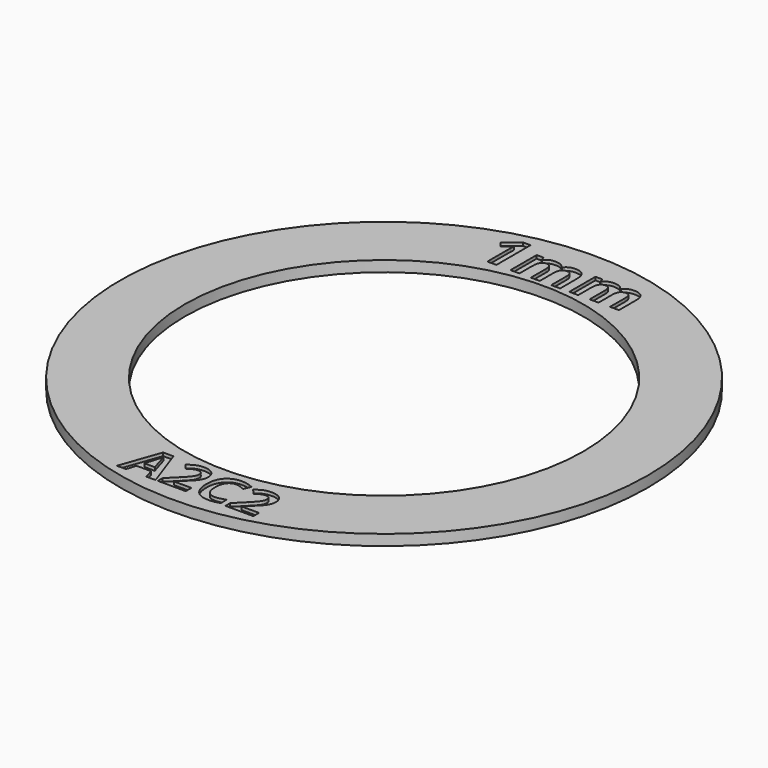
from build123d import *

# Parameters (mm, degrees)
F0_R           = 24.5
F0_R_2         = 18.5
F0_TEXT_SIZE   = 5.1974965673
F0_TEXT_SIZE_2 = 5.5555555556
F1_DEPTH       = 1
F2_DEPTH       = 0.3


# Not quite as in the source:
# - Text() gives the source's letters only with a copy of the font that has no kerning and outlines rounded to 1/6400 em; it was checked with that copy


with BuildPart() as f1:
    # F0 (on Top) → F1 (new body)
    with BuildSketch(Plane.XY):
        Circle(F0_R)
        Polygon((-2.9154707307, -22.8730905801), (-3.7633123583, -22.8730905801), (-4.0321203839, -21.9895161637), (-5.3850937091, -21.9895161637), (-5.6539017347, -22.8730905801), (-6.5017433622, -22.8730905801), (-5.1918118055, -19.1471352284), (-4.2302749405, -19.1471352284), align=None, mode=Mode.SUBTRACT)
        with BuildLine():
            Line((-0.1136952374, -22.2128460943), (-0.1136952374, -22.8730905801))
            Line((-0.1136952374, -22.8730905801), (-2.707570868, -22.8730905801))
            Line((-2.707570868, -22.8730905801), (-2.707570868, -22.3273534405))
            Line((-2.707570868, -22.3273534405), (-1.7760820301, -21.3861192965))
            add(Edge.make_bspline(
                [(-1.7760820301, -21.3861192965), (-1.3619065224, -20.9621984828), (-1.2352175436, -20.7985585518)],
                knots=[0, 0, 0, 1, 1, 1], degree=2))
            add(Edge.make_bspline(
                [(-1.2352175436, -20.7985585518), (-1.1085285648, -20.6349186208), (-1.0524930549, -20.4952359005)],
                knots=[0, 0, 0, 1, 1, 1], degree=2))
            add(Edge.make_bspline(
                [(-1.0524930549, -20.4952359005), (-0.996457545, -20.3555531803), (-0.996457545, -20.206125154)],
                knots=[0, 0, 0, 1, 1, 1], degree=2))
            add(Edge.make_bspline(
                [(-0.996457545, -20.206125154), (-0.996457545, -19.9827952234), (-1.1198980885, -19.8735665846)],
                knots=[0, 0, 0, 1, 1, 1], degree=2))
            add(Edge.make_bspline(
                [(-1.1198980885, -19.8735665846), (-1.243338632, -19.7643379458), (-1.4488021681, -19.7643379458)],
                knots=[0, 0, 0, 1, 1, 1], degree=2))
            add(Edge.make_bspline(
                [(-1.4488021681, -19.7643379458), (-1.6640110104, -19.7643379458), (-1.86703822, -19.8634152241)],
                knots=[0, 0, 0, 1, 1, 1], degree=2))
            add(Edge.make_bspline(
                [(-1.86703822, -19.8634152241), (-2.0700654297, -19.9624925024), (-2.2909590338, -20.1452169911)],
                knots=[0, 0, 0, 1, 1, 1], degree=2))
            Line((-2.2909590338, -20.1452169911), (-2.7173161741, -19.6400852935))
            add(Edge.make_bspline(
                [(-2.7173161741, -19.6400852935), (-2.4436354955, -19.4061979479), (-2.2633473333, -19.3099630505)],
                knots=[0, 0, 0, 1, 1, 1], degree=2))
            add(Edge.make_bspline(
                [(-2.2633473333, -19.3099630505), (-2.0830591711, -19.2137281532), (-1.869880601, -19.1617531875)],
                knots=[0, 0, 0, 1, 1, 1], degree=2))
            add(Edge.make_bspline(
                [(-1.869880601, -19.1617531875), (-1.6567020308, -19.1097782218), (-1.3927666583, -19.1097782218)],
                knots=[0, 0, 0, 1, 1, 1], degree=2))
            add(Edge.make_bspline(
                [(-1.3927666583, -19.1097782218), (-1.0451840753, -19.1097782218), (-0.7788123763, -19.2364672006)],
                knots=[0, 0, 0, 1, 1, 1], degree=2))
            add(Edge.make_bspline(
                [(-0.7788123763, -19.2364672006), (-0.5124406772, -19.3631561795), (-0.365042923, -19.5917648176)],
                knots=[0, 0, 0, 1, 1, 1], degree=2))
            add(Edge.make_bspline(
                [(-0.365042923, -19.5917648176), (-0.2176451688, -19.8203734556), (-0.2176451688, -20.1143568552)],
                knots=[0, 0, 0, 1, 1, 1], degree=2))
            add(Edge.make_bspline(
                [(-0.2176451688, -20.1143568552), (-0.2176451688, -20.3709832482), (-0.3077892498, -20.5955313421)],
                knots=[0, 0, 0, 1, 1, 1], degree=2))
            add(Edge.make_bspline(
                [(-0.3077892498, -20.5955313421), (-0.3979333309, -20.820079436), (-0.5871546903, -21.0559970536)],
                knots=[0, 0, 0, 1, 1, 1], degree=2))
            add(Edge.make_bspline(
                [(-0.5871546903, -21.0559970536), (-0.7763760497, -21.2919146713), (-1.253083938, -21.7288292265)],
                knots=[0, 0, 0, 1, 1, 1], degree=2))
            Line((-1.253083938, -21.7288292265), (-1.7306039352, -22.1779254142))
            Line((-1.7306039352, -22.1779254142), (-1.7306039352, -22.2128460943))
            Line((-1.7306039352, -22.2128460943), (-0.1136952374, -22.2128460943))
        make_face(mode=Mode.SUBTRACT)
        Circle(F0_R_2, mode=Mode.SUBTRACT)
        with BuildLine():
            add(Edge.make_bspline(
                [(2.5077920937, -19.8378337957), (2.2974559045, -19.7643379458), (2.0944286949, -19.7643379458)],
                knots=[0, 0, 0, 1, 1, 1], degree=2))
            add(Edge.make_bspline(
                [(2.0944286949, -19.7643379458), (1.6502051601, -19.7643379458), (1.4065725085, -20.0981146785)],
                knots=[0, 0, 0, 1, 1, 1], degree=2))
            add(Edge.make_bspline(
                [(1.4065725085, -20.0981146785), (1.1629398569, -20.4318914111), (1.1629398569, -21.0279792987)],
                knots=[0, 0, 0, 1, 1, 1], degree=2))
            add(Edge.make_bspline(
                [(1.1629398569, -21.0279792987), (1.1629398569, -22.2688816042), (2.0944286949, -22.2688816042)],
                knots=[0, 0, 0, 1, 1, 1], degree=2))
            add(Edge.make_bspline(
                [(2.0944286949, -22.2688816042), (2.4850530463, -22.2688816042), (3.0405354919, -22.0739754829)],
                knots=[0, 0, 0, 1, 1, 1], degree=2))
            Line((3.0405354919, -22.0739754829), (3.0405354919, -22.7334078599))
            add(Edge.make_bspline(
                [(3.0405354919, -22.7334078599), (2.5841303246, -22.9242534369), (2.0205267906, -22.9242534369)],
                knots=[0, 0, 0, 1, 1, 1], degree=2))
            add(Edge.make_bspline(
                [(2.0205267906, -22.9242534369), (1.2108542784, -22.9242534369), (0.7820608116, -22.4329275896)],
                knots=[0, 0, 0, 1, 1, 1], degree=2))
            add(Edge.make_bspline(
                [(0.7820608116, -22.4329275896), (0.3532673448, -21.9416017422), (0.3532673448, -21.0231066457)],
                knots=[0, 0, 0, 1, 1, 1], degree=2))
            add(Edge.make_bspline(
                [(0.3532673448, -21.0231066457), (0.3532673448, -20.4440730437), (0.5640095884, -20.0087827062)],
                knots=[0, 0, 0, 1, 1, 1], degree=2))
            add(Edge.make_bspline(
                [(0.5640095884, -20.0087827062), (0.7747518321, -19.5734923687), (1.1694367277, -19.3416352953)],
                knots=[0, 0, 0, 1, 1, 1], degree=2))
            add(Edge.make_bspline(
                [(1.1694367277, -19.3416352953), (1.5641216232, -19.1097782218), (2.0944286949, -19.1097782218)],
                knots=[0, 0, 0, 1, 1, 1], degree=2))
            add(Edge.make_bspline(
                [(2.0944286949, -19.1097782218), (2.6344810726, -19.1097782218), (3.1802182121, -19.370465159)],
                knots=[0, 0, 0, 1, 1, 1], degree=2))
            Line((3.1802182121, -19.370465159), (2.9268402545, -20.0104069239))
            add(Edge.make_bspline(
                [(2.9268402545, -20.0104069239), (2.7181282829, -19.9113296456), (2.5077920937, -19.8378337957)],
                knots=[0, 0, 0, 1, 1, 1], degree=2))
        make_face(mode=Mode.SUBTRACT)
        with BuildLine():
            Line((6.1647181942, -22.2128460943), (6.1647181942, -22.8730905801))
            Line((6.1647181942, -22.8730905801), (3.5708425635, -22.8730905801))
            Line((3.5708425635, -22.8730905801), (3.5708425635, -22.3273534405))
            Line((3.5708425635, -22.3273534405), (4.5023314015, -21.3861192965))
            add(Edge.make_bspline(
                [(4.5023314015, -21.3861192965), (4.9165069092, -20.9621984828), (5.043195888, -20.7985585518)],
                knots=[0, 0, 0, 1, 1, 1], degree=2))
            add(Edge.make_bspline(
                [(5.043195888, -20.7985585518), (5.1698848668, -20.6349186208), (5.2259203767, -20.4952359005)],
                knots=[0, 0, 0, 1, 1, 1], degree=2))
            add(Edge.make_bspline(
                [(5.2259203767, -20.4952359005), (5.2819558866, -20.3555531803), (5.2819558866, -20.206125154)],
                knots=[0, 0, 0, 1, 1, 1], degree=2))
            add(Edge.make_bspline(
                [(5.2819558866, -20.206125154), (5.2819558866, -19.9827952234), (5.1585153431, -19.8735665846)],
                knots=[0, 0, 0, 1, 1, 1], degree=2))
            add(Edge.make_bspline(
                [(5.1585153431, -19.8735665846), (5.0350747996, -19.7643379458), (4.8296112634, -19.7643379458)],
                knots=[0, 0, 0, 1, 1, 1], degree=2))
            add(Edge.make_bspline(
                [(4.8296112634, -19.7643379458), (4.6144024212, -19.7643379458), (4.4113752115, -19.8634152241)],
                knots=[0, 0, 0, 1, 1, 1], degree=2))
            add(Edge.make_bspline(
                [(4.4113752115, -19.8634152241), (4.2083480019, -19.9624925024), (3.9874543978, -20.1452169911)],
                knots=[0, 0, 0, 1, 1, 1], degree=2))
            Line((3.9874543978, -20.1452169911), (3.5610972575, -19.6400852935))
            add(Edge.make_bspline(
                [(3.5610972575, -19.6400852935), (3.8347779361, -19.4061979479), (4.0150660983, -19.3099630505)],
                knots=[0, 0, 0, 1, 1, 1], degree=2))
            add(Edge.make_bspline(
                [(4.0150660983, -19.3099630505), (4.1953542604, -19.2137281532), (4.4085328306, -19.1617531875)],
                knots=[0, 0, 0, 1, 1, 1], degree=2))
            add(Edge.make_bspline(
                [(4.4085328306, -19.1617531875), (4.6217114007, -19.1097782218), (4.8856467733, -19.1097782218)],
                knots=[0, 0, 0, 1, 1, 1], degree=2))
            add(Edge.make_bspline(
                [(4.8856467733, -19.1097782218), (5.2332293562, -19.1097782218), (5.4996010553, -19.2364672006)],
                knots=[0, 0, 0, 1, 1, 1], degree=2))
            add(Edge.make_bspline(
                [(5.4996010553, -19.2364672006), (5.7659727544, -19.3631561795), (5.9133705086, -19.5917648176)],
                knots=[0, 0, 0, 1, 1, 1], degree=2))
            add(Edge.make_bspline(
                [(5.9133705086, -19.5917648176), (6.0607682628, -19.8203734556), (6.0607682628, -20.1143568552)],
                knots=[0, 0, 0, 1, 1, 1], degree=2))
            add(Edge.make_bspline(
                [(6.0607682628, -20.1143568552), (6.0607682628, -20.3709832482), (5.9706241817, -20.5955313421)],
                knots=[0, 0, 0, 1, 1, 1], degree=2))
            add(Edge.make_bspline(
                [(5.9706241817, -20.5955313421), (5.8804801006, -20.820079436), (5.6912587412, -21.0559970536)],
                knots=[0, 0, 0, 1, 1, 1], degree=2))
            add(Edge.make_bspline(
                [(5.6912587412, -21.0559970536), (5.5020373818, -21.2919146713), (5.0253294935, -21.7288292265)],
                knots=[0, 0, 0, 1, 1, 1], degree=2))
            Line((5.0253294935, -21.7288292265), (4.5478094964, -22.1779254142))
            Line((4.5478094964, -22.1779254142), (4.5478094964, -22.2128460943))
            Line((4.5478094964, -22.2128460943), (6.1647181942, -22.2128460943))
        make_face(mode=Mode.SUBTRACT)
        with BuildLine():
            Line((-4.7178819444, 22.8950881169), (-4.7178819444, 18.9289422836))
            Line((-4.7178819444, 18.9289422836), (-5.5564236111, 18.9289422836))
            Line((-5.5564236111, 18.9289422836), (-5.5564236111, 21.2240811725))
            Line((-5.5564236111, 21.2240811725), (-5.5477430556, 21.6008172836))
            Line((-5.5477430556, 21.6008172836), (-5.5347222222, 22.0131436725))
            add(Edge.make_bspline(
                [(-5.5347222222, 22.0131436725), (-5.7430555556, 21.8048103392), (-5.8246527778, 21.7397061725)],
                knots=[0, 0, 0, 1, 1, 1], degree=2))
            Line((-5.8246527778, 21.7397061725), (-6.2803819444, 21.3733867281))
            Line((-6.2803819444, 21.3733867281), (-6.6848958333, 21.8777270058))
            Line((-6.6848958333, 21.8777270058), (-5.4071180556, 22.8950881169))
            Line((-5.4071180556, 22.8950881169), (-4.7178819444, 22.8950881169))
        make_face(mode=Mode.SUBTRACT)
        with BuildLine():
            Line((-0.6927083333, 20.4506436725), (-0.6927083333, 18.9289422836))
            Line((-0.6927083333, 18.9289422836), (-1.5199652778, 18.9289422836))
            Line((-1.5199652778, 18.9289422836), (-1.5199652778, 20.7006436725))
            add(Edge.make_bspline(
                [(-1.5199652778, 20.7006436725), (-1.5199652778, 21.0287686725), (-1.6297743056, 21.1928311725)],
                knots=[0, 0, 0, 1, 1, 1], degree=2))
            add(Edge.make_bspline(
                [(-1.6297743056, 21.1928311725), (-1.7395833333, 21.3568936725), (-1.9756944444, 21.3568936725)],
                knots=[0, 0, 0, 1, 1, 1], degree=2))
            add(Edge.make_bspline(
                [(-1.9756944444, 21.3568936725), (-2.2934027778, 21.3568936725), (-2.4370659722, 21.1233867281)],
                knots=[0, 0, 0, 1, 1, 1], degree=2))
            add(Edge.make_bspline(
                [(-2.4370659722, 21.1233867281), (-2.5807291667, 20.8898797836), (-2.5807291667, 20.3560256169)],
                knots=[0, 0, 0, 1, 1, 1], degree=2))
            Line((-2.5807291667, 20.3560256169), (-2.5807291667, 18.9289422836))
            Line((-2.5807291667, 18.9289422836), (-3.4079861111, 18.9289422836))
            Line((-3.4079861111, 18.9289422836), (-3.4079861111, 21.9619283947))
            Line((-3.4079861111, 21.9619283947), (-2.7760416667, 21.9619283947))
            Line((-2.7760416667, 21.9619283947), (-2.6649305556, 21.5739075614))
            Line((-2.6649305556, 21.5739075614), (-2.6189236111, 21.5739075614))
            add(Edge.make_bspline(
                [(-2.6189236111, 21.5739075614), (-2.4965277778, 21.7831089503), (-2.2660590278, 21.9007304781)],
                knots=[0, 0, 0, 1, 1, 1], degree=2))
            add(Edge.make_bspline(
                [(-2.2660590278, 21.9007304781), (-2.0355902778, 22.0183520058), (-1.7369791667, 22.0183520058)],
                knots=[0, 0, 0, 1, 1, 1], degree=2))
            add(Edge.make_bspline(
                [(-1.7369791667, 22.0183520058), (-1.0564236111, 22.0183520058), (-0.8142361111, 21.5739075614)],
                knots=[0, 0, 0, 1, 1, 1], degree=2))
            Line((-0.8142361111, 21.5739075614), (-0.7413194444, 21.5739075614))
            add(Edge.make_bspline(
                [(-0.7413194444, 21.5739075614), (-0.6189236111, 21.7857131169), (-0.3819444444, 21.9020325614)],
                knots=[0, 0, 0, 1, 1, 1], degree=2))
            add(Edge.make_bspline(
                [(-0.3819444444, 21.9020325614), (-0.1449652778, 22.0183520058), (0.1536458333, 22.0183520058)],
                knots=[0, 0, 0, 1, 1, 1], degree=2))
            add(Edge.make_bspline(
                [(0.1536458333, 22.0183520058), (0.6692708333, 22.0183520058), (0.93359375, 21.7540290892)],
                knots=[0, 0, 0, 1, 1, 1], degree=2))
            add(Edge.make_bspline(
                [(0.93359375, 21.7540290892), (1.1979166667, 21.4897061725), (1.1979166667, 20.9063728392)],
                knots=[0, 0, 0, 1, 1, 1], degree=2))
            Line((1.1979166667, 20.9063728392), (1.1979166667, 18.9289422836))
            Line((1.1979166667, 18.9289422836), (0.3680555556, 18.9289422836))
            Line((0.3680555556, 18.9289422836), (0.3680555556, 20.7006436725))
            add(Edge.make_bspline(
                [(0.3680555556, 20.7006436725), (0.3680555556, 21.0287686725), (0.2582465278, 21.1928311725)],
                knots=[0, 0, 0, 1, 1, 1], degree=2))
            add(Edge.make_bspline(
                [(0.2582465278, 21.1928311725), (0.1484375, 21.3568936725), (-0.0876736111, 21.3568936725)],
                knots=[0, 0, 0, 1, 1, 1], degree=2))
            add(Edge.make_bspline(
                [(-0.0876736111, 21.3568936725), (-0.3914930556, 21.3568936725), (-0.5421006944, 21.1398797836)],
                knots=[0, 0, 0, 1, 1, 1], degree=2))
            add(Edge.make_bspline(
                [(-0.5421006944, 21.1398797836), (-0.6927083333, 20.9228658947), (-0.6927083333, 20.4506436725)],
                knots=[0, 0, 0, 1, 1, 1], degree=2))
        make_face(mode=Mode.SUBTRACT)
        with BuildLine():
            Line((4.7621527778, 20.4506436725), (4.7621527778, 18.9289422836))
            Line((4.7621527778, 18.9289422836), (3.9348958333, 18.9289422836))
            Line((3.9348958333, 18.9289422836), (3.9348958333, 20.7006436725))
            add(Edge.make_bspline(
                [(3.9348958333, 20.7006436725), (3.9348958333, 21.0287686725), (3.8250868056, 21.1928311725)],
                knots=[0, 0, 0, 1, 1, 1], degree=2))
            add(Edge.make_bspline(
                [(3.8250868056, 21.1928311725), (3.7152777778, 21.3568936725), (3.4791666667, 21.3568936725)],
                knots=[0, 0, 0, 1, 1, 1], degree=2))
            add(Edge.make_bspline(
                [(3.4791666667, 21.3568936725), (3.1614583333, 21.3568936725), (3.0177951389, 21.1233867281)],
                knots=[0, 0, 0, 1, 1, 1], degree=2))
            add(Edge.make_bspline(
                [(3.0177951389, 21.1233867281), (2.8741319444, 20.8898797836), (2.8741319444, 20.3560256169)],
                knots=[0, 0, 0, 1, 1, 1], degree=2))
            Line((2.8741319444, 20.3560256169), (2.8741319444, 18.9289422836))
            Line((2.8741319444, 18.9289422836), (2.046875, 18.9289422836))
            Line((2.046875, 18.9289422836), (2.046875, 21.9619283947))
            Line((2.046875, 21.9619283947), (2.6788194444, 21.9619283947))
            Line((2.6788194444, 21.9619283947), (2.7899305556, 21.5739075614))
            Line((2.7899305556, 21.5739075614), (2.8359375, 21.5739075614))
            add(Edge.make_bspline(
                [(2.8359375, 21.5739075614), (2.9583333333, 21.7831089503), (3.1888020833, 21.9007304781)],
                knots=[0, 0, 0, 1, 1, 1], degree=2))
            add(Edge.make_bspline(
                [(3.1888020833, 21.9007304781), (3.4192708333, 22.0183520058), (3.7178819444, 22.0183520058)],
                knots=[0, 0, 0, 1, 1, 1], degree=2))
            add(Edge.make_bspline(
                [(3.7178819444, 22.0183520058), (4.3984375, 22.0183520058), (4.640625, 21.5739075614)],
                knots=[0, 0, 0, 1, 1, 1], degree=2))
            Line((4.640625, 21.5739075614), (4.7135416667, 21.5739075614))
            add(Edge.make_bspline(
                [(4.7135416667, 21.5739075614), (4.8359375, 21.7857131169), (5.0729166667, 21.9020325614)],
                knots=[0, 0, 0, 1, 1, 1], degree=2))
            add(Edge.make_bspline(
                [(5.0729166667, 21.9020325614), (5.3098958333, 22.0183520058), (5.6085069444, 22.0183520058)],
                knots=[0, 0, 0, 1, 1, 1], degree=2))
            add(Edge.make_bspline(
                [(5.6085069444, 22.0183520058), (6.1241319444, 22.0183520058), (6.3884548611, 21.7540290892)],
                knots=[0, 0, 0, 1, 1, 1], degree=2))
            add(Edge.make_bspline(
                [(6.3884548611, 21.7540290892), (6.6527777778, 21.4897061725), (6.6527777778, 20.9063728392)],
                knots=[0, 0, 0, 1, 1, 1], degree=2))
            Line((6.6527777778, 20.9063728392), (6.6527777778, 18.9289422836))
            Line((6.6527777778, 18.9289422836), (5.8229166667, 18.9289422836))
            Line((5.8229166667, 18.9289422836), (5.8229166667, 20.7006436725))
            add(Edge.make_bspline(
                [(5.8229166667, 20.7006436725), (5.8229166667, 21.0287686725), (5.7131076389, 21.1928311725)],
                knots=[0, 0, 0, 1, 1, 1], degree=2))
            add(Edge.make_bspline(
                [(5.7131076389, 21.1928311725), (5.6032986111, 21.3568936725), (5.3671875, 21.3568936725)],
                knots=[0, 0, 0, 1, 1, 1], degree=2))
            add(Edge.make_bspline(
                [(5.3671875, 21.3568936725), (5.0633680556, 21.3568936725), (4.9127604167, 21.1398797836)],
                knots=[0, 0, 0, 1, 1, 1], degree=2))
            add(Edge.make_bspline(
                [(4.9127604167, 21.1398797836), (4.7621527778, 20.9228658947), (4.7621527778, 20.4506436725)],
                knots=[0, 0, 0, 1, 1, 1], degree=2))
        make_face(mode=Mode.SUBTRACT)
        with Locations((-6.5017433622, -22.8730905801)):
            Text('A2C2', F0_TEXT_SIZE, font='Open Sans', font_style=FontStyle.BOLD, text_align=(TextAlign.LEFT, TextAlign.BOTTOM))
        with Locations((-7.0130208333, 18.9289422836)):
            Text('1mm', F0_TEXT_SIZE_2, font='Open Sans', font_style=FontStyle.BOLD, text_align=(TextAlign.LEFT, TextAlign.BOTTOM))
        with BuildLine():
            Line((-5.1869391524, -21.3300837867), (-4.2205296344, -21.3300837867))
            add(Edge.make_bspline(
                [(-4.2205296344, -21.3300837867), (-4.5932875914, -20.1297869232), (-4.640389904, -19.9722378085)],
                knots=[0, 0, 0, 1, 1, 1], degree=2))
            add(Edge.make_bspline(
                [(-4.640389904, -19.9722378085), (-4.6874922167, -19.8146886938), (-4.7077949376, -19.7237325038)],
                knots=[0, 0, 0, 1, 1, 1], degree=2))
            add(Edge.make_bspline(
                [(-4.7077949376, -19.7237325038), (-4.791442148, -20.0485760393), (-5.1869391524, -21.3300837867)],
                knots=[0, 0, 0, 1, 1, 1], degree=2))
        make_face()
    extrude(amount=-F1_DEPTH)

    # F0 (on Top) → F2 (cut)
    with BuildSketch(Plane.XY):
        with Locations((-6.5017433622, -22.8730905801)):
            Text('A2C2', F0_TEXT_SIZE, font='Open Sans', font_style=FontStyle.BOLD, text_align=(TextAlign.LEFT, TextAlign.BOTTOM))
        with Locations((-7.0130208333, 18.9289422836)):
            Text('1mm', F0_TEXT_SIZE_2, font='Open Sans', font_style=FontStyle.BOLD, text_align=(TextAlign.LEFT, TextAlign.BOTTOM))
    extrude(amount=-F2_DEPTH, mode=Mode.SUBTRACT)


solid = f1.part
